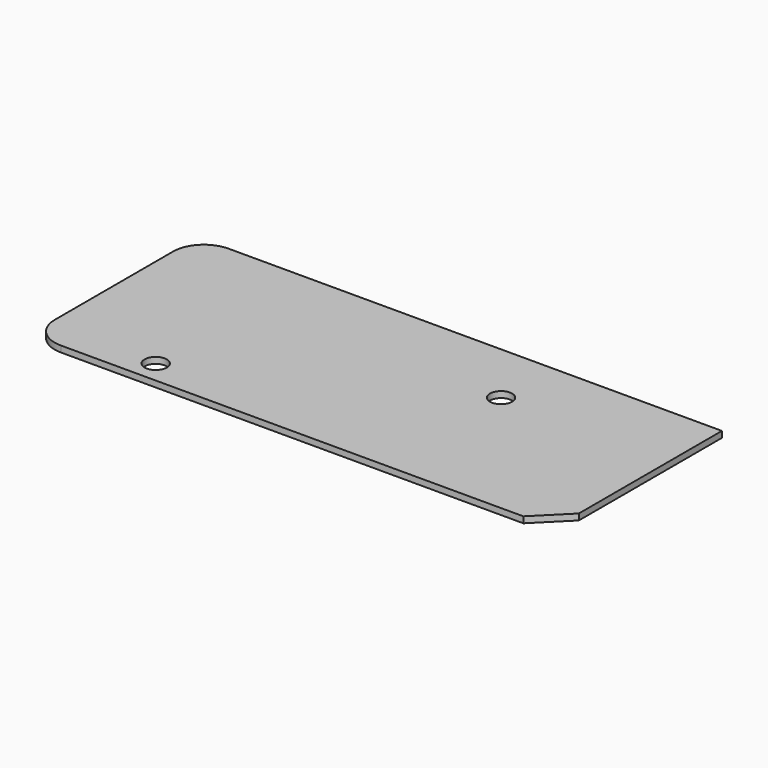
from build123d import *

# Parameters (mm, degrees)
F1_DEPTH = 1
F3_D     = 3.6
F4_SIZE  = 5


with BuildPart() as f1:
    # F0 (on Top) → F1 (new body)
    with BuildSketch(Plane.XY):
        with BuildLine():
            Line((41.9170247219, -17.6387755275), (41.9170247219, 16.3612244725))
            Line((41.9170247219, 16.3612244725), (-38.0829752781, 16.3612244725))
            ThreePointArc((-38.0829752781, 16.3612244725), (-41.618509184, 14.8967583785), (-43.0829752781, 11.3612244725))
            Line((-43.0829752781, 11.3612244725), (-43.0829752781, -12.6387755275))
            ThreePointArc((-43.0829752781, -12.6387755275), (-41.618509184, -16.1743094334), (-38.0829752781, -17.6387755275))
            Line((-38.0829752781, -17.6387755275), (41.9170247219, -17.6387755275))
        make_face()
    extrude(amount=F1_DEPTH)

    # F3 (through all)
    with Locations(Plane(origin=(0, 0, 0), x_dir=(1, 0, 0), z_dir=(0, 0, -1))):
        with Locations((-25.6229752781, 13.9887755275), (14.3770247219, -6.0112244725)):
            Hole(F3_D / 2)

    # F4
    f4_edges = [f1.edges().sort_by_distance(p)[0] for p in [
        (41.917025, -17.638776, 0.5),
    ]]
    chamfer(f4_edges, length=F4_SIZE)


solid = f1.part
